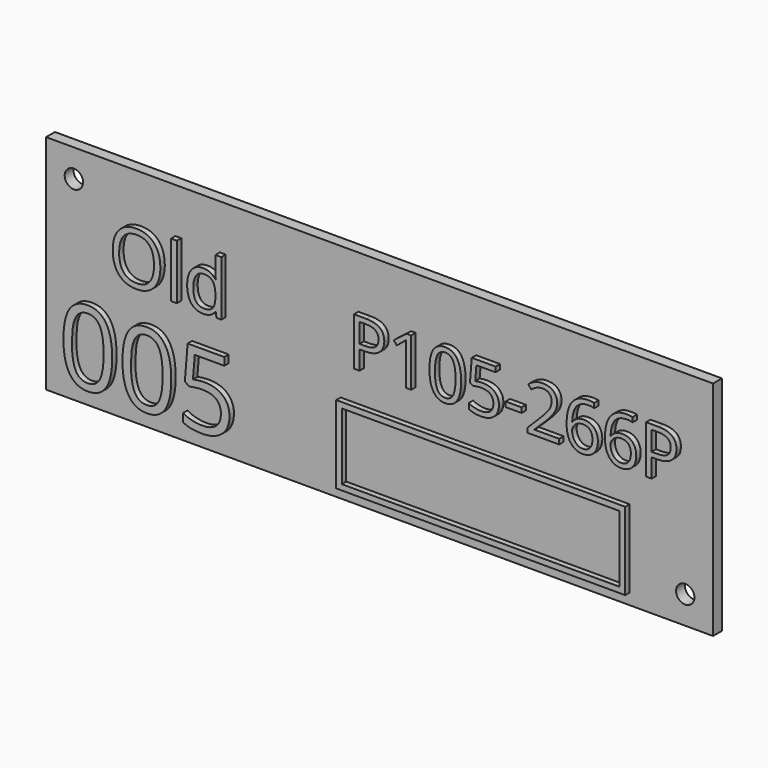
from build123d import *

# Parameters (mm, degrees)
F0_W          = 120
F0_H          = 40
F1_DEPTH      = 2
F3_D          = 3.3
F4_TEXT_SIZE  = 12.073193737
F5_DEPTH      = 1
F6_TEXT_SIZE  = 18.5776487663
F7_DEPTH      = 1
F8_W          = 52
F8_H          = 14
F8_W_2        = 49.99999962
F8_H_2        = 11.99999962
F9_DEPTH      = 1
F10_TEXT_SIZE = 13.0388495579
F11_DEPTH     = 1


# Not quite as in the source:
# - Text() gives the source's letters only with a copy of the font that has no kerning and outlines rounded to 1/6400 em; it was checked with that copy


with BuildPart() as f1:
    # F0 (on Front) → F1 (new body)
    with BuildSketch(Plane.XZ):
        Rectangle(F0_W, F0_H)
    extrude(amount=F1_DEPTH)

    # F3 (through all)
    with Locations(Plane.XZ.offset(2)):
        with Locations((-55, 15), (55, -15)):
            Hole(F3_D / 2)

    # F4 (on face) → F5 (join)
    with BuildSketch(Plane.XZ.offset(2)):
        with Locations((-5, 2)):
            Text('P105-266P', F4_TEXT_SIZE, font='Open Sans', text_align=(TextAlign.LEFT, TextAlign.BOTTOM))
    extrude(amount=F5_DEPTH)

    # F6 (on face) → F7 (join)
    with BuildSketch(Plane.XZ.offset(2)):
        with Locations((-57, -17)):
            Text('005', F6_TEXT_SIZE, font='Open Sans', text_align=(TextAlign.LEFT, TextAlign.BOTTOM))
    extrude(amount=F7_DEPTH)

    # F8 (on face) → F9 (join)
    with BuildSketch(Plane.XZ.offset(2)):
        with Locations((19, -11)):
            Rectangle(F8_W, F8_H)
        with Locations((19, -11)):
            Rectangle(F8_W_2, F8_H_2, mode=Mode.SUBTRACT)
    extrude(amount=F9_DEPTH)

    # F10 (on face) → F11 (join)
    with BuildSketch(Plane.XZ.offset(2)):
        with Locations((-48, 2)):
            Text('Old', F10_TEXT_SIZE, font='Open Sans', text_align=(TextAlign.LEFT, TextAlign.BOTTOM))
    extrude(amount=F11_DEPTH)


solid = f1.part
